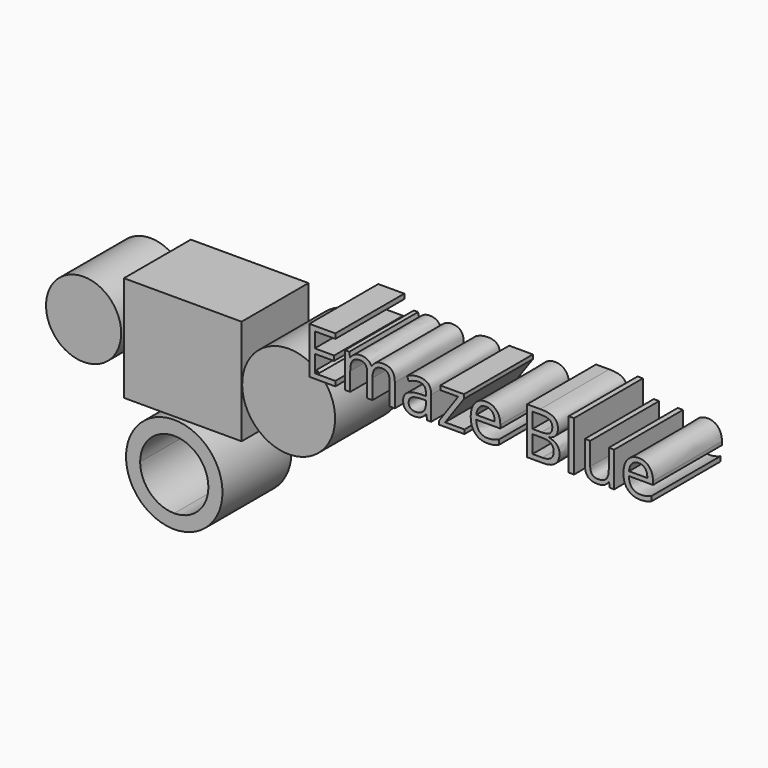
from build123d import *

# Parameters (mm, degrees)
F0_R         = 14.6488168802
F0_TEXT_SIZE = 19.85839982
F1_DEPTH     = 26.162
F2_W         = 35.737156868
F2_H         = 31.9932652637
F3_DEPTH     = 25.4
F4_R         = 14.1195598804
F5_DEPTH     = 25.4
F4_R_2       = 11.4158177249


# Not quite as in the source:
# - Text() gives the source's letters only with a copy of the font that has no kerning and outlines rounded to 1/6400 em; it was checked with that copy


with BuildPart() as f1:
    # F0 (on Front) → F1 (new body)
    with BuildSketch(Plane.XZ):
        Circle(F0_R)
        with BuildLine():
            ThreePointArc((7.746467718, 6.8805076565), (9.6852945524, 3.680246887), (10.3609433797, 0))
            ThreePointArc((10.3609433797, 0), (9.450864986, -4.2462099256), (6.8805076565, -7.746467718))
            ThreePointArc((6.8805076565, -7.746467718), (3.680246887, -9.6852945524), (0, -10.3609433797))
            ThreePointArc((0, -10.3609433797), (-7.3262933233, -7.3262933233), (-10.3609433797, 0))
            ThreePointArc((-10.3609433797, 0), (-9.450864986, 4.2462099256), (-6.8805076565, 7.746467718))
            ThreePointArc((-6.8805076565, 7.746467718), (-3.680246887, 9.6852945524), (0, 10.3609433797))
            ThreePointArc((0, 10.3609433797), (4.2462099256, 9.450864986), (7.746467718, 6.8805076565))
        make_face(mode=Mode.SUBTRACT)
        with Locations((39.0864368528, 39.4839085639)):
            Text('Emaze Blue', F0_TEXT_SIZE, font='Open Sans', text_align=(TextAlign.LEFT, TextAlign.BOTTOM))
    extrude(amount=F1_DEPTH)

    # F4 (on Front) → F5 (join)
    with BuildSketch(Plane.XZ):
        with Locations((34.1378934681, 30.3457025439)):
            Circle(F4_R)
    extrude(amount=F5_DEPTH)


with BuildPart() as f3:
    # F2 (on Front) → F3 (new body)
    with BuildSketch(Plane.XZ):
        with Locations((1.974452287, 31.0264104046)):
            Rectangle(F2_W, F2_H)
    extrude(amount=F3_DEPTH)


with BuildPart() as f5:
    # F4 (on Front) → F5, piece 2 (new body)
    with BuildSketch(Plane.XZ):
        with Locations((-28.146866709, 32.0474728942)):
            Circle(F4_R_2)
    extrude(amount=F5_DEPTH)


solid = Compound([f1.part, f3.part, f5.part])
